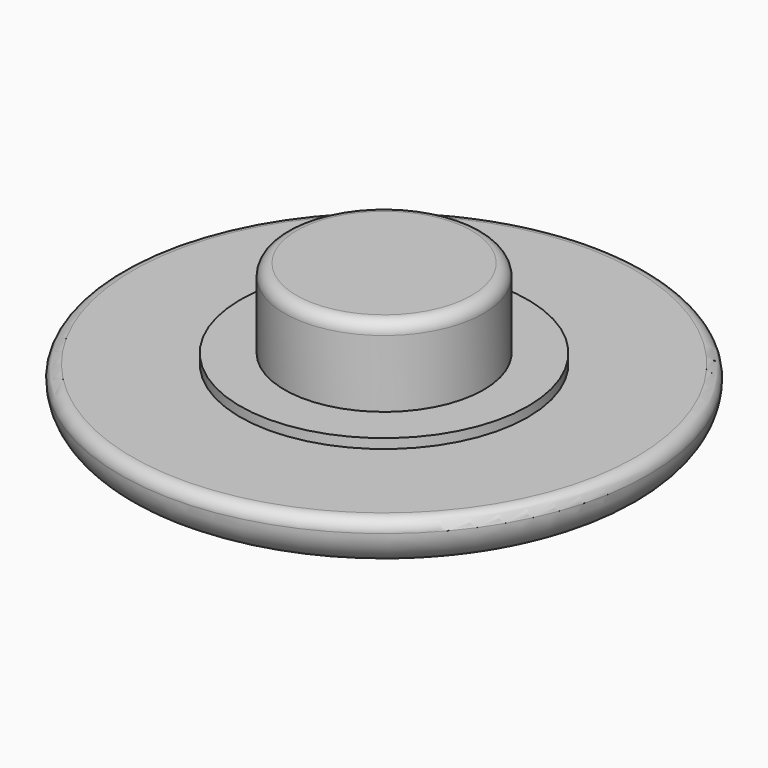
from build123d import *

# Parameters (mm, degrees)
F0_R         = 11
F0_R_2       = 6
F0_R_3       = 4.15
F1_DEPTH     = 2
F2_DEPTH     = 2.4
F3_DEPTH     = 5.7
F4_R         = 0.5
F5_R         = 0.5
F6_R         = 1.49999
F7_TEXT_SIZE = 11.1111111111
F8_DEPTH     = 1


# Not quite as in the source:
# - a fillet or chamfer is up to 0.001 mm smaller than in the source, because OpenCascade refuses the exact size
# - Text() gives the source's letters only with a copy of the font that has no kerning and outlines rounded to 1/6400 em; it was checked with that copy


with BuildPart() as f1:
    # F0 (on Top) → F1 (new body)
    with BuildSketch(Plane.XY):
        Circle(F0_R)
        Circle(F0_R_2, mode=Mode.SUBTRACT)
        Circle(F0_R_2)
        Circle(F0_R_3, mode=Mode.SUBTRACT)
        Circle(F0_R_3)
    extrude(amount=F1_DEPTH)

    # F0 (on Top) → F2 (join)
    with BuildSketch(Plane.XY):
        Circle(F0_R_2)
        Circle(F0_R_3, mode=Mode.SUBTRACT)
    extrude(amount=F2_DEPTH)

    # F0 (on Top) → F3 (join)
    with BuildSketch(Plane.XY):
        Circle(F0_R_3)
    extrude(amount=F3_DEPTH)

    # F4
    f4_edges = [f1.edges().sort_by_distance(p)[0] for p in [
        (-11, 0, 2),
    ]]
    fillet(f4_edges, radius=F4_R)

    # F5
    f5_edges = [f1.edges().sort_by_distance(p)[0] for p in [
        (-4.15, 0, 5.7),
    ]]
    fillet(f5_edges, radius=F5_R)

    # F6 (radius 1.5 in the source; OpenCascade refuses exactly that, so slightly less here)
    f6_edges = [f1.edges().sort_by_distance(p)[0] for p in [
        (-11, 0, 0),
    ]]
    fillet(f6_edges, radius=F6_R)

    # F7 (on face) → F8 (cut)
    with BuildSketch(Plane(origin=(0, 0, 0), x_dir=(1, 0, 0), z_dir=(0, 0, -1))):
        with Locations((-5.0989583333, -4)):
            Text('M', F7_TEXT_SIZE, font='Open Sans', font_style=FontStyle.BOLD, text_align=(TextAlign.LEFT, TextAlign.BOTTOM))
    extrude(amount=-F8_DEPTH, mode=Mode.SUBTRACT)


solid = f1.part
